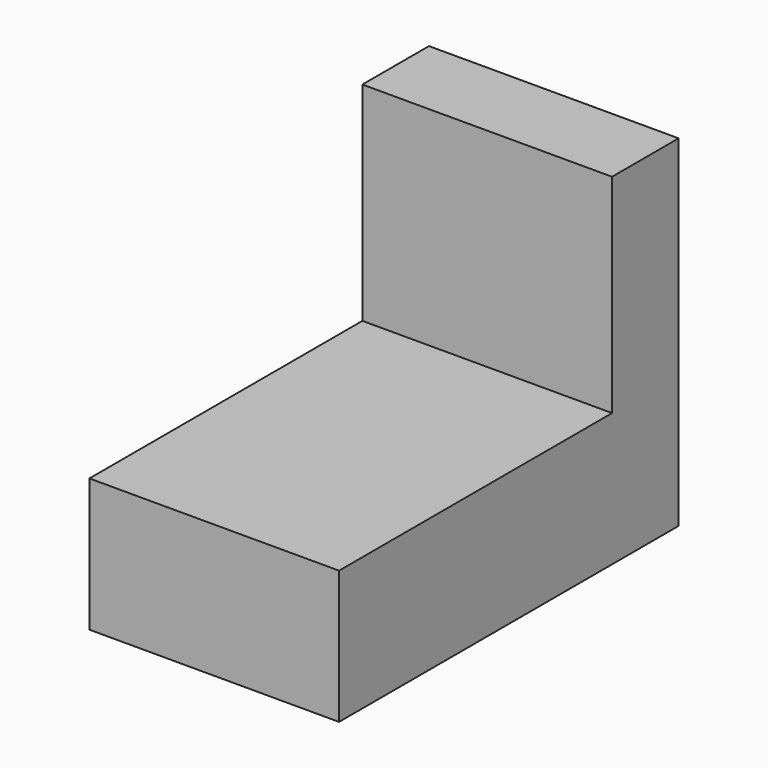
from build123d import *

# Parameters (mm, degrees)
F0_W     = 600
F0_H     = 1020
F1_DEPTH = 820
F2_W     = 600
F2_H     = 820
F3_DEPTH = 500


with BuildPart() as f1:
    # F0 (on Top) → F1 (new body)
    with BuildSketch(Plane.XY):
        Rectangle(F0_W, F0_H)
    extrude(amount=F1_DEPTH)

    # F2 (on face) → F3 (cut)
    with BuildSketch(Plane.XY.offset(820)):
        with Locations((0, -100)):
            Rectangle(F2_W, F2_H)
    extrude(amount=-F3_DEPTH, mode=Mode.SUBTRACT)


solid = f1.part
